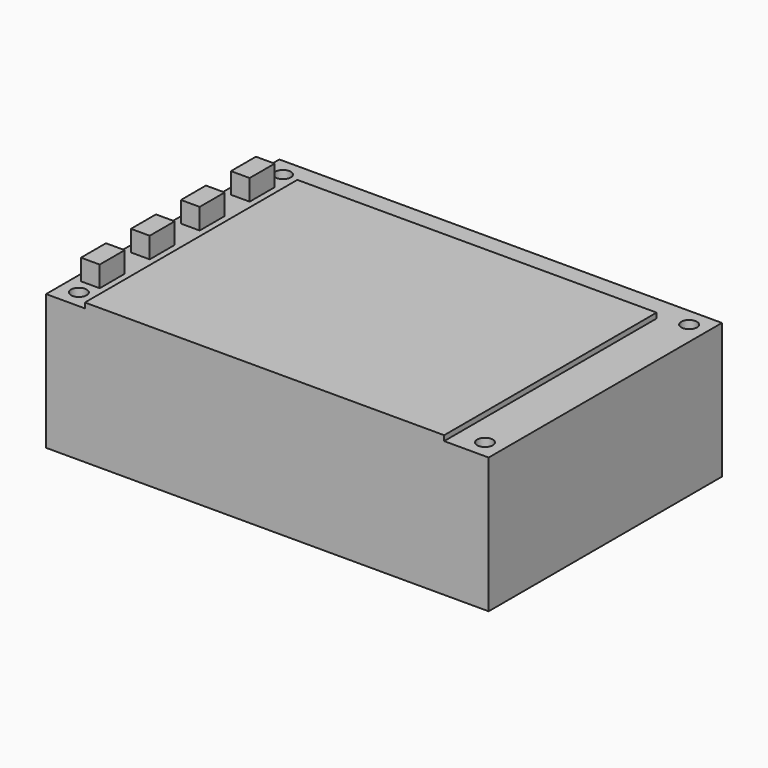
from build123d import *

# Parameters (mm, degrees)
F0_W     = 85
F0_H     = 56
F0_R     = 1.5
F1_DEPTH = 26
F2_W     = 69
F2_H     = 51
F3_DEPTH = 1
F4_W     = 3.6
F4_H     = 6
F5_DEPTH = 4


with BuildPart() as f1:
    # F0 (on Top) → F1 (new body)
    with BuildSketch(Plane.XY):
        with Locations((0, -3.51239704)):
            Rectangle(F0_W, F0_H)
        with Locations((-39, -28.01239704)):
            Circle(F0_R, mode=Mode.SUBTRACT)
        with Locations((39, -28.01239704)):
            Circle(F0_R, mode=Mode.SUBTRACT)
        with Locations((-39, 20.98760296)):
            Circle(F0_R, mode=Mode.SUBTRACT)
        with Locations((39, 20.98760296)):
            Circle(F0_R, mode=Mode.SUBTRACT)
    extrude(amount=F1_DEPTH)

    # F2 (on face) → F3 (join)
    with BuildSketch(Plane.XY.offset(26)):
        with Locations((-0.5440037453, -6.01239704)):
            Rectangle(F2_W, F2_H)
    extrude(amount=F3_DEPTH)

    # F4 (on face) → F5 (join)
    with BuildSketch(Plane.XY.offset(26)):
        with Locations((-39.2, 13.98760296)):
            Rectangle(F4_W, F4_H)
        with Locations((-39.2, 1.98760296)):
            Rectangle(F4_W, F4_H)
        with Locations((-39.2, -10.01239704)):
            Rectangle(F4_W, F4_H)
        with Locations((-39.2, -22.01239704)):
            Rectangle(F4_W, F4_H)
    extrude(amount=F5_DEPTH)


solid = f1.part
